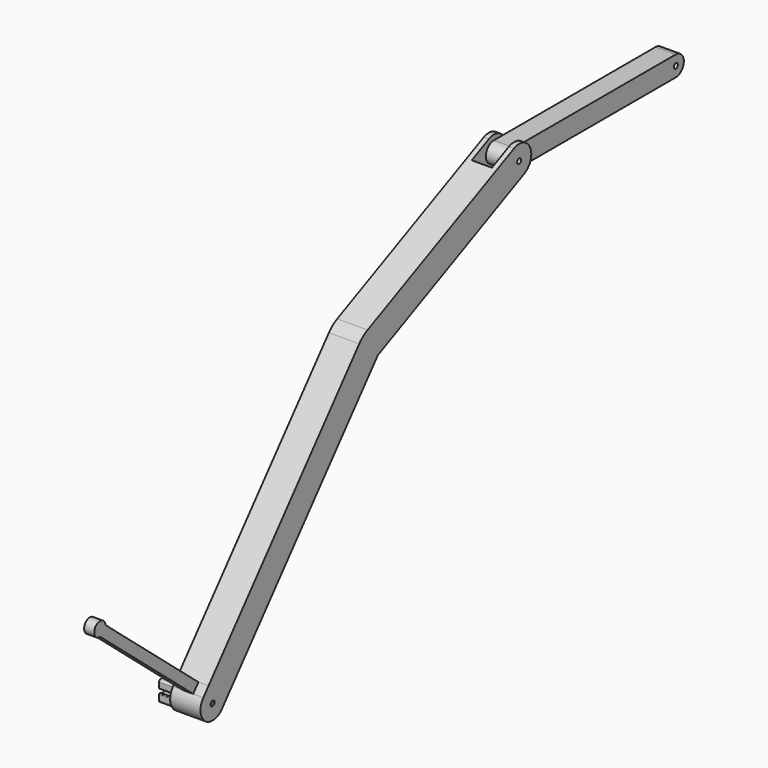
from build123d import *

# Parameters (mm, degrees)
F0_R          = 5
F2_DEPTH      = 30
F4_W          = 40
F4_H          = 60
F5_DEPTH      = 46.5
F5_DEPTH_BACK = 41.1
F1_R          = 5
F6_DEPTH      = 20
F7_R          = 5
F8_DEPTH      = 30
F9_SIZE       = 1
F10_DEPTH     = 10
F11_R         = 3.4


# Not quite as in the source:
# - ends of sketch curves that miss each other by under 0.0002 mm in the source are joined


with BuildPart() as f2:
    # F0 (on Right) → F2 (new body, symmetric)
    with BuildSketch(Plane.YZ):
        with BuildLine():
            Line((-10.1255810998, 34.604517153), (-22.9813332936, 19.2836282906))
            ThreePointArc((-22.9813332936, 19.2836282906), (-19.2836282906, -22.9813332936), (22.9813332936, -19.2836282906))
            Line((22.9813332936, -19.2836282906), (408.6538991055, 440.3430375808))
            Line((408.6538991055, 440.3430375808), (771.1770139202, 609.3903422771))
            ThreePointArc((771.1770139202, 609.3903422771), (785.687699679, 649.2581237404), (745.8199182157, 663.7688094993))
            Line((745.8199182157, 663.7688094993), (383.2968034011, 494.721504803))
            ThreePointArc((383.2968034011, 494.721504803), (372.128213365, 487.9442379983), (362.6912325184, 478.910294162))
            Line((362.6912325184, 478.910294162), (-10.1255810998, 34.604517153))
        make_face()
        Circle(F0_R, mode=Mode.SUBTRACT)
        with Locations((758.4984660679, 636.5795758882)):
            Circle(F0_R, mode=Mode.SUBTRACT)
    extrude(amount=F2_DEPTH, both=True)

    # F4 (on 3pt) → F5 (cut, two sides)
    with BuildSketch(Plane(origin=(0, 866.8500643674, 404.2188234867), x_dir=(1, 0, 0), z_dir=(0, -0.906307787, -0.4226182617))) as f5_sk:
        with Locations((0, 256.3817234333)):
            Rectangle(F4_W, F4_H)
    extrude(amount=F5_DEPTH, mode=Mode.SUBTRACT)
    extrude(f5_sk.sketch, amount=-F5_DEPTH_BACK, mode=Mode.SUBTRACT)

    # F0 (on Right) → F10 (join, symmetric)
    with BuildSketch(Plane.YZ):
        with BuildLine():
            Line((-252.7946662293, 212.1199111966), (-22.9813332936, 19.2836282906))
            Line((-22.9813332936, 19.2836282906), (-10.1255810998, 34.604517153))
            Line((-10.1255810998, 34.604517153), (-239.9389140355, 227.4408000589))
            ThreePointArc((-239.9389140355, 227.4408000589), (-264.5970843598, 235.0773887902), (-252.7946662293, 212.1199111966))
        make_face()
    extrude(amount=F10_DEPTH, both=True)


with BuildPart() as f6:
    # F1 (on Right) → F6 (new body, symmetric)
    with BuildSketch(Plane.YZ):
        with BuildLine():
            Line((1158.4984660679, 656.5795758882), (758.4984660679, 656.5795758882))
            ThreePointArc((758.4984660679, 656.5795758882), (738.4984660679, 636.5795758882), (758.4984660679, 616.5795758882))
            Line((758.4984660679, 616.5795758882), (1158.4984660679, 616.5795758882))
            ThreePointArc((1158.4984660679, 616.5795758882), (1178.4984660679, 636.5795758882), (1158.4984660679, 656.5795758882))
        make_face()
        with BuildLine():
            ThreePointArc((758.4984660679, 641.5795758882), (762.0339999739, 640.1151097941), (763.4984660679, 636.5795758882))
            ThreePointArc((763.4984660679, 636.5795758882), (754.962932162, 633.0440419822), (758.4984660679, 641.5795758882))
        make_face(mode=Mode.SUBTRACT)
        with Locations((1158.4984660679, 636.5795758882)):
            Circle(F1_R, mode=Mode.SUBTRACT)
    extrude(amount=F6_DEPTH, both=True)


with BuildPart() as f8:
    # F7 (on Right) → F8 (new body, symmetric)
    with BuildSketch(Plane.YZ):
        Circle(F7_R)
    extrude(amount=F8_DEPTH, both=True)

    # F9
    f9_edges = [f8.edges().sort_by_distance(p)[0] for p in [
        (-30, -5, 0),
        (30, -5, 0),
    ]]
    chamfer(f9_edges, length=F9_SIZE)


with BuildPart() as f13:
    # F13: sweep along a path in F12
    with BuildLine(Plane.XY) as f13_path:
        Line((0, 0), (-59.893, 0))
    # F11 (on Right) → F13 (sweep)
    with BuildSketch(Plane.YZ):
        with BuildLine():
            ThreePointArc((-20, -16), (-18.8284271247, -18.8284271247), (-16, -20))
            Line((-16, -20), (-5.5, -20))
            ThreePointArc((-5.5, -20), (-4.4393398282, -19.5606601718), (-4, -18.5))
            Line((-4, -18.5), (-4, -16.5))
            ThreePointArc((-4, -16.5), (-4.2928932188, -15.7928932188), (-5, -15.5))
            Line((-5, -15.5), (-6.75, -15.5))
            ThreePointArc((-6.75, -15.5), (-6.9267766953, -15.5732233047), (-7, -15.75))
            Line((-7, -15.75), (-7, -17.75))
            ThreePointArc((-7, -17.75), (-7.0732233047, -17.9267766953), (-7.25, -18))
            Line((-7.25, -18), (-7.5, -18))
            ThreePointArc((-7.5, -18), (-9.267766953, -17.267766953), (-10, -15.5))
            Line((-10, -15.5), (-10, -14.72036))
            ThreePointArc((-10, -14.72036), (-9.8959912568, -14.0837933075), (-9.594782846, -13.5134351166))
            ThreePointArc((-9.594782846, -13.5134351166), (-7.2640297924, -10.8489962236), (-4.5803049475, -8.5404760706))
            ThreePointArc((-4.5803049475, -8.5404760706), (-3.4504153043, -7.9527578982), (-2.193056, -7.75))
            Line((-2.193056, -7.75), (2.193056, -7.75))
            ThreePointArc((2.193056, -7.75), (3.4504153043, -7.9527578982), (4.5803048437, -8.5404762101))
            ThreePointArc((4.5803048437, -8.5404762101), (7.2640297924, -10.8489962236), (9.5947827328, -13.5134352022))
            ThreePointArc((9.5947827328, -13.5134352022), (9.8959912568, -14.0837933075), (10, -14.72036))
            Line((10, -14.72036), (10, -15.5))
            ThreePointArc((10, -15.5), (9.267766953, -17.267766953), (7.5, -18))
            Line((7.5, -18), (7.25, -18))
            ThreePointArc((7.25, -18), (7.0732233047, -17.9267766953), (7, -17.75))
            Line((7, -17.75), (7, -15.75))
            ThreePointArc((7, -15.75), (6.9267766953, -15.5732233047), (6.75, -15.5))
            Line((6.75, -15.5), (5, -15.5))
            ThreePointArc((5, -15.5), (4.2928932188, -15.7928932188), (4, -16.5))
            Line((4, -16.5), (4, -18.5))
            ThreePointArc((4, -18.5), (4.4393398282, -19.5606601718), (5.5, -20))
            Line((5.5, -20), (16, -20))
            ThreePointArc((16, -20), (18.8284271247, -18.8284271247), (20, -16))
            Line((20, -16), (20, -5.5))
            ThreePointArc((20, -5.5), (19.5606601718, -4.4393398282), (18.5, -4))
            Line((18.5, -4), (16.5, -4))
            ThreePointArc((16.5, -4), (15.7928932188, -4.2928932188), (15.5, -5))
            Line((15.5, -5), (15.5, -6.75))
            ThreePointArc((15.5, -6.75), (15.5732233047, -6.9267766953), (15.75, -7))
            Line((15.75, -7), (17.75, -7))
            ThreePointArc((17.75, -7), (17.9267766953, -7.0732233047), (18, -7.25))
            Line((18, -7.25), (18, -7.5))
            ThreePointArc((18, -7.5), (17.267766953, -9.267766953), (15.5, -10))
            Line((15.5, -10), (14.72036, -10))
            ThreePointArc((14.72036, -10), (14.0837930214, -9.8959911608), (13.5134346354, -9.5947824818))
            ThreePointArc((13.5134346354, -9.5947824818), (10.8489962236, -7.2640297924), (8.5404760706, -4.5803049475))
            ThreePointArc((8.5404760706, -4.5803049475), (7.9527578982, -3.4504153043), (7.75, -2.193056))
            Line((7.75, -2.193056), (7.75, 2.193056))
            ThreePointArc((7.75, 2.193056), (7.9527578982, 3.4504153043), (8.5404762101, 4.5803048437))
            ThreePointArc((8.5404762101, 4.5803048437), (10.8489962236, 7.2640297924), (13.5134352022, 9.5947827328))
            ThreePointArc((13.5134352022, 9.5947827328), (14.0837933075, 9.8959912568), (14.72036, 10))
            Line((14.72036, 10), (15.5, 10))
            ThreePointArc((15.5, 10), (17.267766953, 9.267766953), (18, 7.5))
            Line((18, 7.5), (18, 7.25))
            ThreePointArc((18, 7.25), (17.9267766953, 7.0732233047), (17.75, 7))
            Line((17.75, 7), (15.75, 7))
            ThreePointArc((15.75, 7), (15.5732233047, 6.9267766953), (15.5, 6.75))
            Line((15.5, 6.75), (15.5, 5))
            ThreePointArc((15.5, 5), (15.7928932188, 4.2928932188), (16.5, 4))
            Line((16.5, 4), (18.5, 4))
            ThreePointArc((18.5, 4), (19.5606601718, 4.4393398282), (20, 5.5))
            Line((20, 5.5), (20, 16))
            ThreePointArc((20, 16), (18.8284271247, 18.8284271247), (16, 20))
            Line((16, 20), (5.5, 20))
            ThreePointArc((5.5, 20), (4.4393398282, 19.5606601718), (4, 18.5))
            Line((4, 18.5), (4, 16.5))
            ThreePointArc((4, 16.5), (4.2928932188, 15.7928932188), (5, 15.5))
            Line((5, 15.5), (6.75, 15.5))
            ThreePointArc((6.75, 15.5), (6.9267766953, 15.5732233047), (7, 15.75))
            Line((7, 15.75), (7, 17.75))
            ThreePointArc((7, 17.75), (7.0732233047, 17.9267766953), (7.25, 18))
            Line((7.25, 18), (7.5, 18))
            ThreePointArc((7.5, 18), (9.267766953, 17.267766953), (10, 15.5))
            Line((10, 15.5), (10, 14.72036))
            ThreePointArc((10, 14.72036), (9.8959910339, 14.0837926435), (9.5947820006, 13.5134339995))
            ThreePointArc((9.5947820006, 13.5134339995), (7.2640295093, 10.8489959429), (4.5803049475, 8.5404760706))
            ThreePointArc((4.5803049475, 8.5404760706), (3.4504153043, 7.9527578982), (2.193056, 7.75))
            Line((2.193056, 7.75), (-2.193056, 7.75))
            ThreePointArc((-2.193056, 7.75), (-3.4504153043, 7.9527578982), (-4.5803048437, 8.5404762101))
            ThreePointArc((-4.5803048437, 8.5404762101), (-7.2640297924, 10.8489962236), (-9.5947827328, 13.5134352022))
            ThreePointArc((-9.5947827328, 13.5134352022), (-9.8959912568, 14.0837933075), (-10, 14.72036))
            Line((-10, 14.72036), (-10, 15.5))
            ThreePointArc((-10, 15.5), (-9.267766953, 17.267766953), (-7.5, 18))
            Line((-7.5, 18), (-7.25, 18))
            ThreePointArc((-7.25, 18), (-7.0732233047, 17.9267766953), (-7, 17.75))
            Line((-7, 17.75), (-7, 15.75))
            ThreePointArc((-7, 15.75), (-6.9267766953, 15.5732233047), (-6.75, 15.5))
            Line((-6.75, 15.5), (-5, 15.5))
            ThreePointArc((-5, 15.5), (-4.2928932188, 15.7928932188), (-4, 16.5))
            Line((-4, 16.5), (-4, 18.5))
            ThreePointArc((-4, 18.5), (-4.4393398282, 19.5606601718), (-5.5, 20))
            Line((-5.5, 20), (-16, 20))
            ThreePointArc((-16, 20), (-18.8284271247, 18.8284271247), (-20, 16))
            Line((-20, 16), (-20, 5.5))
            ThreePointArc((-20, 5.5), (-19.5606601718, 4.4393398282), (-18.5, 4))
            Line((-18.5, 4), (-16.5, 4))
            ThreePointArc((-16.5, 4), (-15.7928932188, 4.2928932188), (-15.5, 5))
            Line((-15.5, 5), (-15.5, 6.75))
            ThreePointArc((-15.5, 6.75), (-15.5732233047, 6.9267766953), (-15.75, 7))
            Line((-15.75, 7), (-17.75, 7))
            ThreePointArc((-17.75, 7), (-17.9267766953, 7.0732233047), (-18, 7.25))
            Line((-18, 7.25), (-18, 7.5))
            ThreePointArc((-18, 7.5), (-17.267766953, 9.267766953), (-15.5, 10))
            Line((-15.5, 10), (-14.72036, 10))
            ThreePointArc((-14.72036, 10), (-14.0837933075, 9.8959912568), (-13.5134351166, 9.594782846))
            ThreePointArc((-13.5134351166, 9.594782846), (-10.8489962236, 7.2640297924), (-8.5404760706, 4.5803049475))
            ThreePointArc((-8.5404760706, 4.5803049475), (-7.9527578982, 3.4504153043), (-7.75, 2.193056))
            Line((-7.75, 2.193056), (-7.75, -2.193056))
            ThreePointArc((-7.75, -2.193056), (-7.9527578982, -3.4504153043), (-8.5404762101, -4.5803048437))
            ThreePointArc((-8.5404762101, -4.5803048437), (-10.8489960111, -7.2640295781), (-13.513434721, -9.5947823686))
            ThreePointArc((-13.513434721, -9.5947823686), (-14.0837926435, -9.8959910339), (-14.72036, -10))
            Line((-14.72036, -10), (-15.5, -10))
            ThreePointArc((-15.5, -10), (-17.267766953, -9.267766953), (-18, -7.5))
            Line((-18, -7.5), (-18, -7.25))
            ThreePointArc((-18, -7.25), (-17.9267766953, -7.0732233047), (-17.75, -7))
            Line((-17.75, -7), (-15.75, -7))
            ThreePointArc((-15.75, -7), (-15.5732233047, -6.9267766953), (-15.5, -6.75))
            Line((-15.5, -6.75), (-15.5, -5))
            ThreePointArc((-15.5, -5), (-15.7928932188, -4.2928932188), (-16.5, -4))
            Line((-16.5, -4), (-18.5, -4))
            ThreePointArc((-18.5, -4), (-19.5606601718, -4.4393398282), (-20, -5.5))
            Line((-20, -5.5), (-20, -16))
        make_face()
        with BuildLine():
            Line((-11.733888, -10.327511), (-10.327177, -11.734221))
            ThreePointArc((-10.327177, -11.734221), (-10.1816471856, -12.0575358414), (-10.2870795422, -12.3960555754))
            Line((-10.2870795422, -12.3960555754), (-10.551319, -12.739281))
            ThreePointArc((-10.551319, -12.739281), (-11.0332530301, -13.6518533492), (-11.199667, -14.67036))
            Line((-11.199667, -14.67036), (-11.199667, -18.299999))
            ThreePointArc((-11.199667, -18.299999), (-11.3461132559, -18.653553037), (-11.699667, -18.8))
            Line((-11.699667, -18.8), (-15.999667, -18.799999))
            ThreePointArc((-15.999667, -18.799999), (-17.9795659873, -17.9798989873), (-18.799667, -16))
            Line((-18.799667, -16), (-18.799667, -11.700001))
            ThreePointArc((-18.799667, -11.700001), (-18.6532207441, -11.346446963), (-18.299667, -11.2))
            Line((-18.299667, -11.2), (-14.670027, -11.200001))
            ThreePointArc((-14.670027, -11.200001), (-13.6515200631, -11.0335859341), (-12.7389468016, -10.5516522622))
            Line((-12.7389468016, -10.5516522622), (-12.395722, -10.287411))
            ThreePointArc((-12.395722, -10.287411), (-12.0572020803, -10.1819792299), (-11.733888, -10.327511))
        make_face(mode=Mode.SUBTRACT)
        with BuildLine():
            ThreePointArc((-8.8828102271, -10.7476507897), (-9.2400711188, -10.9078191023), (-9.6032096835, -10.7614646835))
            Line((-9.6032096835, -10.7614646835), (-10.761465, -9.60321))
            ThreePointArc((-10.761465, -9.60321), (-10.9078191023, -9.2400711188), (-10.7476507897, -8.8828102271))
            ThreePointArc((-10.7476507897, -8.8828102271), (-9.0898525604, -7.2025956354), (-7.59, -5.38))
            ThreePointArc((-7.59, -5.38), (-6.9342622771, -4.2218027894), (-6.594007615, -2.9350870504))
            ThreePointArc((-6.594007615, -2.9350870504), (-6.4280439456, -2.6241972621), (-6.098239, -2.500001))
            Line((-6.098239, -2.500001), (-4.609773, -2.5))
            ThreePointArc((-4.609773, -2.5), (-4.3714066692, -2.5604752919), (-4.1907021902, -2.7272721238))
            ThreePointArc((-4.1907021902, -2.7272721238), (-3.5355339059, -3.5355339059), (-2.7272717711, -4.1907026483))
            ThreePointArc((-2.7272717711, -4.1907026483), (-2.5604754002, -4.3714064694), (-2.5, -4.609771))
            Line((-2.5, -4.609771), (-2.5, -6.09824))
            ThreePointArc((-2.5, -6.09824), (-2.6241968403, -6.4280449811), (-2.935086949, -6.5940073893))
            ThreePointArc((-2.935086949, -6.5940073893), (-4.2218031598, -6.934262428), (-5.38, -7.59))
            ThreePointArc((-5.38, -7.59), (-7.2025956354, -9.0898525604), (-8.8828102271, -10.7476507897))
        make_face(mode=Mode.SUBTRACT)
        with BuildLine():
            ThreePointArc((11.2, -14.670027), (11.0335857112, -13.6515193991), (10.5516514168, -12.7389456845))
            Line((10.5516514168, -12.7389456845), (10.287411, -12.395721))
            ThreePointArc((10.287411, -12.395721), (10.1819792085, -12.0572024332), (10.3275101094, -11.7338881094))
            Line((10.3275101094, -11.7338881094), (11.734221, -10.327177))
            ThreePointArc((11.734221, -10.327177), (12.0575354485, -10.1816472094), (12.3960549556, -10.2870790567))
            Line((12.3960549556, -10.2870790567), (12.739281, -10.551319))
            ThreePointArc((12.739281, -10.551319), (13.6518533492, -11.0332530301), (14.67036, -11.199667))
            Line((14.67036, -11.199667), (18.299999, -11.199667))
            ThreePointArc((18.299999, -11.199667), (18.653553037, -11.3461132559), (18.8, -11.699667))
            Line((18.8, -11.699667), (18.799999, -15.999668))
            ThreePointArc((18.799999, -15.999668), (17.9798989873, -17.9795659873), (16, -18.799667))
            Line((16, -18.799667), (11.700001, -18.799667))
            ThreePointArc((11.700001, -18.799667), (11.3464473165, -18.6532210977), (11.2, -18.299668))
            Line((11.2, -18.299668), (11.2, -14.670027))
        make_face(mode=Mode.SUBTRACT)
        with BuildLine():
            ThreePointArc((4.1907024877, -2.7272716666), (4.3714064694, -2.5604754002), (4.609771, -2.5))
            Line((4.609771, -2.5), (6.09824, -2.5))
            ThreePointArc((6.09824, -2.5), (6.4280449811, -2.6241968403), (6.5940073893, -2.935086949))
            ThreePointArc((6.5940073893, -2.935086949), (6.934262428, -4.2218031598), (7.59, -5.38))
            ThreePointArc((7.59, -5.38), (9.0898523595, -7.2025954126), (10.7476512045, -8.8828087792))
            ThreePointArc((10.7476512045, -8.8828087792), (10.907819109, -9.2400714723), (10.7614641835, -9.6032101835))
            Line((10.7614641835, -9.6032101835), (9.60321, -10.761465))
            ThreePointArc((9.60321, -10.761465), (9.2400711188, -10.9078191023), (8.8828102271, -10.7476507897))
            ThreePointArc((8.8828102271, -10.7476507897), (7.2025959079, -9.089852806), (5.38, -7.59))
            ThreePointArc((5.38, -7.59), (4.2218027894, -6.9342622771), (2.9350870504, -6.594007615))
            ThreePointArc((2.9350870504, -6.594007615), (2.6241975919, -6.4280443214), (2.500001, -6.09824))
            Line((2.500001, -6.09824), (2.5, -4.609772))
            ThreePointArc((2.5, -4.609772), (2.5604755302, -4.3714062297), (2.7272721238, -4.1907021902))
            ThreePointArc((2.7272721238, -4.1907021902), (3.5355339059, -3.5355339059), (4.1907024877, -2.7272716666))
        make_face(mode=Mode.SUBTRACT)
        with BuildLine():
            Line((-4.609773, 2.5), (-6.098239, 2.5))
            ThreePointArc((-6.098239, 2.5), (-6.4280446053, 2.6241965105), (-6.5940073893, 2.935086949))
            ThreePointArc((-6.5940073893, 2.935086949), (-6.934262428, 4.2218031598), (-7.59, 5.38))
            ThreePointArc((-7.59, 5.38), (-9.0898525604, 7.2025956354), (-10.7476512045, 8.8828087792))
            ThreePointArc((-10.7476512045, 8.8828087792), (-10.9078191023, 9.2400711188), (-10.7614646835, 9.6032096835))
            Line((-10.7614646835, 9.6032096835), (-9.603209, 10.761465))
            ThreePointArc((-9.603209, 10.761465), (-9.2400711188, 10.9078191023), (-8.8828102271, 10.7476507897))
            ThreePointArc((-8.8828102271, 10.7476507897), (-7.2025956354, 9.0898525604), (-5.38, 7.59))
            ThreePointArc((-5.38, 7.59), (-4.2218031598, 6.934262428), (-2.9350870504, 6.594007615))
            ThreePointArc((-2.9350870504, 6.594007615), (-2.6241972621, 6.4280439456), (-2.500001, 6.098239))
            Line((-2.500001, 6.098239), (-2.5, 4.609773))
            ThreePointArc((-2.5, 4.609773), (-2.5604752919, 4.3714066692), (-2.7272721238, 4.1907021902))
            ThreePointArc((-2.7272721238, 4.1907021902), (-3.5355339059, 3.5355339059), (-4.1907026483, 2.7272717711))
            ThreePointArc((-4.1907026483, 2.7272717711), (-4.3714069089, 2.5604751618), (-4.609773, 2.5))
        make_face(mode=Mode.SUBTRACT)
        with BuildLine():
            Line((-10.551652, 12.738946), (-10.287411, 12.395722))
            ThreePointArc((-10.287411, 12.395722), (-10.1819792299, 12.0572020803), (-10.3275106094, 11.7338876094))
            Line((-10.3275106094, 11.7338876094), (-11.734221, 10.327177))
            ThreePointArc((-11.734221, 10.327177), (-12.0575354485, 10.1816472094), (-12.3960549556, 10.2870790567))
            Line((-12.3960549556, 10.2870790567), (-12.73928, 10.551319))
            ThreePointArc((-12.73928, 10.551319), (-13.6518530631, 11.0332529341), (-14.67036, 11.199667))
            Line((-14.67036, 11.199667), (-18.3, 11.199667))
            ThreePointArc((-18.3, 11.199667), (-18.6535533906, 11.3461136094), (-18.8, 11.699667))
            Line((-18.8, 11.699667), (-18.8, 15.999667))
            ThreePointArc((-18.8, 15.999667), (-17.9798989873, 17.9795659873), (-16, 18.799667))
            Line((-16, 18.799667), (-11.7, 18.799667))
            ThreePointArc((-11.7, 18.799667), (-11.3464466094, 18.6532203906), (-11.2, 18.299667))
            Line((-11.2, 18.299667), (-11.2, 14.670027))
            ThreePointArc((-11.2, 14.670027), (-11.0335859341, 13.6515200631), (-10.551652, 12.738946))
        make_face(mode=Mode.SUBTRACT)
        Circle(F11_R, mode=Mode.SUBTRACT)
        with BuildLine():
            Line((9.60321, 10.761465), (10.761465, 9.603209))
            ThreePointArc((10.761465, 9.603209), (10.9078191023, 9.2400711188), (10.7476507897, 8.8828102271))
            ThreePointArc((10.7476507897, 8.8828102271), (9.089852806, 7.2025959079), (7.59, 5.38))
            ThreePointArc((7.59, 5.38), (6.934262428, 4.2218031598), (6.594007615, 2.9350870504))
            ThreePointArc((6.594007615, 2.9350870504), (6.4280443214, 2.6241975919), (6.09824, 2.500001))
            Line((6.09824, 2.500001), (4.609772, 2.5))
            ThreePointArc((4.609772, 2.5), (4.3714062297, 2.5604755302), (4.1907021902, 2.7272721238))
            ThreePointArc((4.1907021902, 2.7272721238), (3.5355339059, 3.5355339059), (2.7272717711, 4.1907026483))
            ThreePointArc((2.7272717711, 4.1907026483), (2.5604751618, 4.3714069089), (2.5, 4.609772))
            Line((2.5, 4.609772), (2.5, 6.098239))
            ThreePointArc((2.5, 6.098239), (2.6241965105, 6.4280446053), (2.935086949, 6.5940073893))
            ThreePointArc((2.935086949, 6.5940073893), (4.2218031598, 6.934262428), (5.38, 7.59))
            ThreePointArc((5.38, 7.59), (7.2025954126, 9.0898523595), (8.8828087792, 10.7476512045))
            ThreePointArc((8.8828087792, 10.7476512045), (9.2400714723, 10.907819109), (9.60321, 10.761465))
        make_face(mode=Mode.SUBTRACT)
        with BuildLine():
            ThreePointArc((12.3957220867, 10.2874108893), (12.0572024332, 10.1819792085), (11.7338881094, 10.3275101094))
            Line((11.7338881094, 10.3275101094), (10.327177, 11.734221))
            ThreePointArc((10.327177, 11.734221), (10.1816472281, 12.0575351408), (10.2870786766, 12.3960544701))
            Line((10.2870786766, 12.3960544701), (10.551319, 12.73928))
            ThreePointArc((10.551319, 12.73928), (11.0332529341, 13.6518530631), (11.199667, 14.67036))
            Line((11.199667, 14.67036), (11.199667, 18.3))
            ThreePointArc((11.199667, 18.3), (11.3461136094, 18.6535533906), (11.699667, 18.8))
            Line((11.699667, 18.8), (15.999668, 18.8))
            ThreePointArc((15.999668, 18.8), (17.9795663409, 17.9798986338), (18.799667, 16))
            Line((18.799667, 16), (18.799667, 11.7))
            ThreePointArc((18.799667, 11.7), (18.6532207441, 11.346446963), (18.299668, 11.2))
            Line((18.299668, 11.2), (14.670029, 11.2))
            ThreePointArc((14.670029, 11.2), (13.6515203471, 11.0335860294), (12.7389456845, 10.5516514168))
            Line((12.7389456845, 10.5516514168), (12.3957220867, 10.2874108893))
        make_face(mode=Mode.SUBTRACT)
    sweep(path=f13_path.line)


solid = Compound([f2.part, f6.part, f8.part, f13.part])
